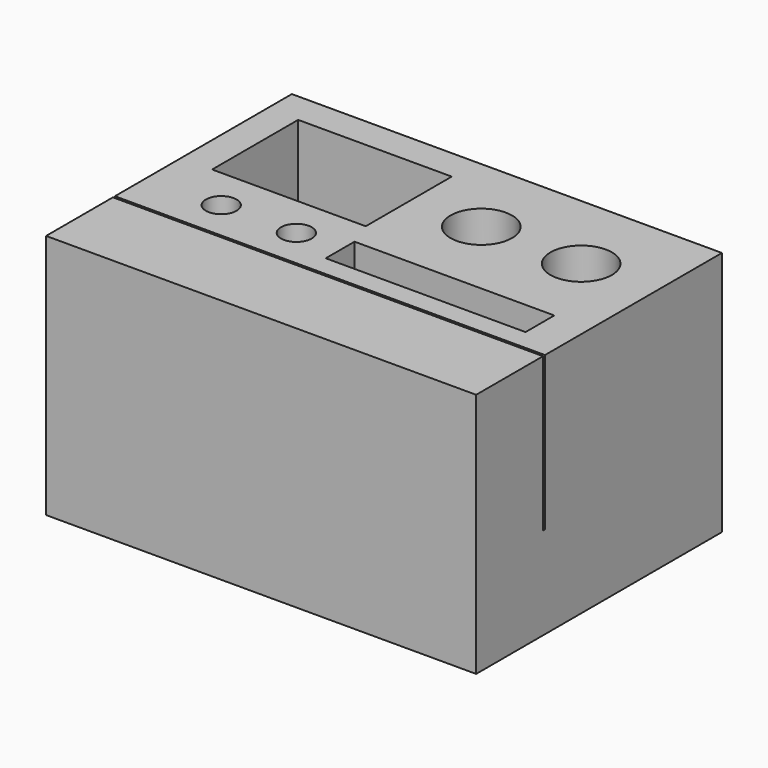
from build123d import *

# Parameters (mm, degrees)
F0_W         = 140
F0_H         = 100
F1_DEPTH     = 80
F2_W         = 140
F2_H         = 0.8107870817
F2_W_2       = 50
F2_H_2       = 35
F2_R         = 10
F2_R_2       = 5
F2_W_3       = 65.0366321206
F2_H_3       = 11.7065925151
F4_DEPTH     = 50
F5_TEXT_SIZE = 14.5833318432
F6_DEPTH     = 15


# Not quite as in the source:
# - the program builds the solid bodies; features that only make, move or delete a surface that nothing else refers to are left out
# - Text() gives the source's letters only with a copy of the font that has no kerning and outlines rounded to 1/6400 em; it was checked with that copy


with BuildPart() as f1:
    # F0 (on Top) → F1 (new body)
    with BuildSketch(Plane.XY):
        with Locations((38.3864191175, 35.6129800901)):
            Rectangle(F0_W, F0_H)
    extrude(amount=F1_DEPTH)

    # F2 (on face) → F4 (cut)
    with BuildSketch(Plane.XY.offset(80)):
        with Locations((38.3864191175, 13.2116600871)):
            Rectangle(F2_W, F2_H)
        with Locations((3.5088489205, 58.0208432674)):
            Rectangle(F2_W_2, F2_H_2)
        with Locations((51.6170337796, 58.6533807218)):
            Circle(F2_R)
        with Locations((84.1353535652, 58.6533807218)):
            Circle(F2_R)
        with Locations((-7.4362298474, 26.6553554684)):
            Circle(F2_R_2)
        with Locations((17.0175451785, 26.6553554684)):
            Circle(F2_R_2)
        with Locations((64.1040690243, 26.2651359662)):
            Rectangle(F2_W_3, F2_H_3)
    extrude(amount=-F4_DEPTH, mode=Mode.SUBTRACT)

    # F5 (on face) → F6 (join)
    with BuildSketch(Plane.XZ.offset(14.3870199099)):
        with Locations((-22.4431548268, 45.9318198264)):
            Text('ADMINISTRATIVO', F5_TEXT_SIZE, font='Open Sans', font_style=FontStyle.BOLD, text_align=(TextAlign.LEFT, TextAlign.BOTTOM))
        with Locations((-7.2856042922, 26.0984885196)):
            Text('IES RODEIRA', F5_TEXT_SIZE, font='Open Sans', font_style=FontStyle.BOLD, text_align=(TextAlign.LEFT, TextAlign.BOTTOM))
    extrude(amount=-F6_DEPTH)


solid = f1.part
